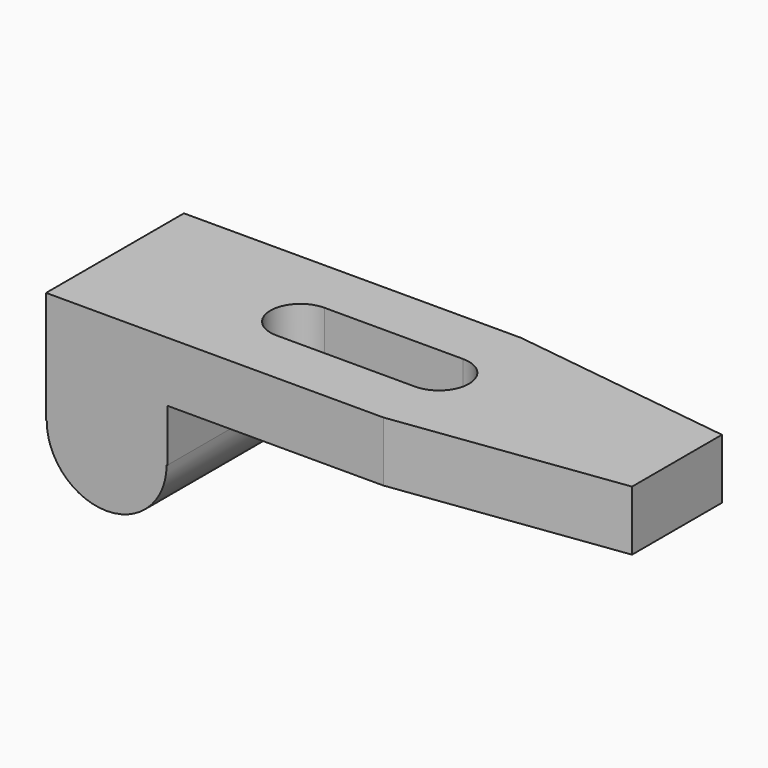
from build123d import *

# Parameters (mm, degrees)
F1_DEPTH = 46
F3_DEPTH = 16
F5_DEPTH = 46.001


# Not quite as in the source:
# - a feature names something its author has since deleted; it is built from what else it names


with BuildPart() as f1:
    # F0 (on Front) → F1 (new body)
    with BuildSketch(Plane.XZ):
        with BuildLine():
            ThreePointArc((0.1762595361, 0), (16.1762595361, -16), (32.1762595361, 0))
            Line((32.1762595361, 0), (0.1762595361, 0))
        make_face()
        with BuildLine():
            Line((0.1762595361, 0), (32.1762595361, 0))
            ThreePointArc((32.1762595361, 0), (16.1762595361, 16), (0.1762595361, 0))
        make_face()
        with BuildLine():
            ThreePointArc((0.1762595361, 0), (16.1762595361, 16), (32.1762595361, 0))
            Line((32.1762595361, 0), (32.3525190723, 0))
            Line((32.3525190723, 0), (32.3525190723, 14))
            Line((32.3525190723, 14), (32.3525190723, 30))
            Line((32.3525190723, 30), (0, 30))
            Line((0, 30), (0, 0))
            Line((0, 0), (0.1762595361, 0))
        make_face()
        Polygon((32.3525190723, 30), (32.3525190723, 14), (150.0428766012, 14), (150.0428766012, 30), (104.9743145704, 30), (67.9628998041, 30), (45.0152419508, 30), align=None)
    extrude(amount=F1_DEPTH)

    # F2 (on face) → F3 (cut)
    with BuildSketch(Plane.XY.offset(30)):
        Polygon((90.0428766012, 0), (150.0428766012, -8), (150.0428766012, 0), align=None)
        Polygon((90.0428766012, -46), (150.0428766012, -46), (150.0428766012, -38), align=None)
    extrude(amount=-F3_DEPTH, mode=Mode.SUBTRACT)

    # F4 (on face) → F5 (cut, through all)
    with BuildSketch(Plane.XY.offset(30)):
        with BuildLine():
            Line((86.5, -15), (68, -15))
            Line((68, -15), (49.5, -15))
            ThreePointArc((49.5, -15), (41.5, -23), (49.5, -31))
            Line((49.5, -31), (68, -31))
            Line((68, -31), (86.5, -31))
            ThreePointArc((86.5, -31), (94.5, -23), (86.5, -15))
        make_face()
    extrude(amount=-F5_DEPTH, mode=Mode.SUBTRACT)


solid = f1.part
